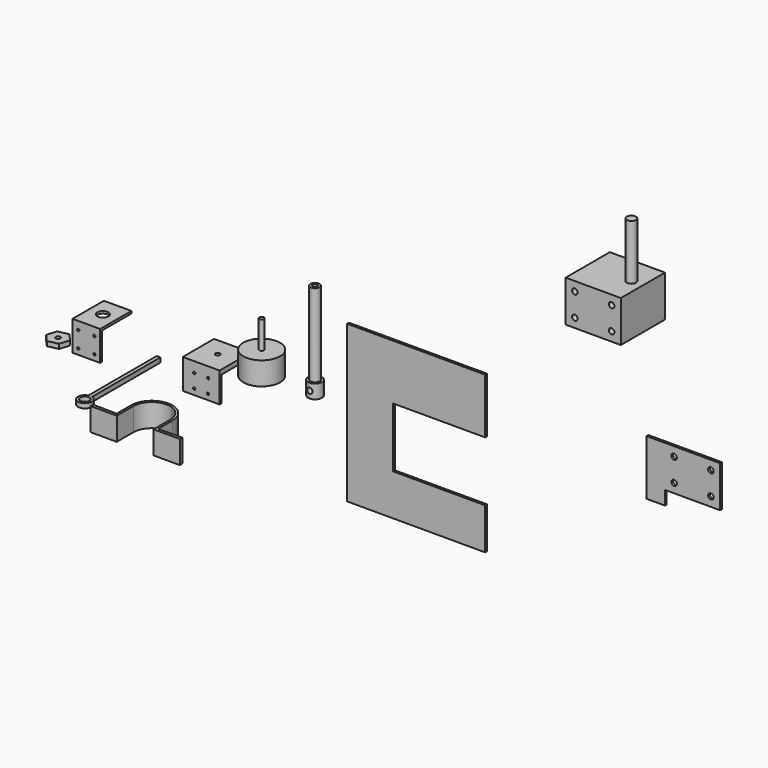
from build123d import *

# Parameters (mm, degrees)
F0_R      = 2.5
F1_DEPTH  = 15
F2_R      = 5
F2_R_2    = 2.5
F3_DEPTH  = 90
F5_R      = 3
F6_DEPTH  = 15.001
F0_R_2    = 20
F7_DEPTH  = 25
F8_R      = 2.5
F9_DEPTH  = 30
F0_W      = 40
F0_H      = 40
F10_DEPTH = 5
F11_W     = 40
F11_H     = 2.5
F12_DEPTH = 32.5
F14_DEPTH = 2.5
F0_W_2    = 30
F0_R_3    = 6
F16_DEPTH = 2.5
F17_W     = 30
F17_H     = 2.5
F18_DEPTH = 32.5
F19_DEPTH = 5
F20_R     = 1.25
F21_DEPTH = 2.5
F22_R     = 1.25
F23_DEPTH = 2.5
F13_W     = 60
F13_H     = 45
F13_R     = 3
F24_DEPTH = 60
F25_R     = 5
F26_DEPTH = 60
F27_DEPTH = 2.5
F28_R     = 3
F29_DEPTH = 25
F0_R_4    = 5
F30_DEPTH = 5
F31_DEPTH = 25


with BuildPart() as f1:
    # F0 (on Top) → F1 (new body)
    with BuildSketch(Plane.XY):
        with BuildLine():
            ThreePointArc((0, 7.5), (-5.3033008589, -5.3033008589), (7.5, 0))
            ThreePointArc((7.5, 0), (5.3033008589, 5.3033008589), (0, 7.5))
        make_face()
        Circle(F0_R, mode=Mode.SUBTRACT)
    extrude(amount=F1_DEPTH)

    # F2 (on face) → F3 (join)
    with BuildSketch(Plane.XY.offset(15)):
        Circle(F2_R)
        Circle(F2_R_2, mode=Mode.SUBTRACT)
    extrude(amount=F3_DEPTH)

    # F5 (on face) → F6 (cut, through all)
    with BuildSketch(Plane.XZ.offset(-7.5)):
        with Locations((0, 7.5)):
            Circle(F5_R)
    extrude(amount=F6_DEPTH, mode=Mode.SUBTRACT)


with BuildPart() as f7:
    # F0 (on Top) → F7 (new body)
    with BuildSketch(Plane.XY):
        with Locations((-57.9745993018, 0)):
            Circle(F0_R_2)
    extrude(amount=F7_DEPTH)

    # F8 (on face) → F9 (join)
    with BuildSketch(Plane.XY.offset(25)):
        with Locations((-57.9745993018, 0)):
            Circle(F8_R)
    extrude(amount=F9_DEPTH)


with BuildPart() as f10:
    # F0 (on Top) → F10 (new body)
    with BuildSketch(Plane.XY):
        with Locations((-105.7388707995, 0)):
            Rectangle(F0_W, F0_H)
        with Locations((-105.7388707995, 0)):
            Circle(F0_R, mode=Mode.SUBTRACT)
    extrude(amount=F10_DEPTH)

    # F11 (on face) → F12 (join)
    with BuildSketch(Plane.XY.offset(5)):
        with Locations((-105.7388707995, -21.25)):
            Rectangle(F11_W, F11_H)
    extrude(amount=-F12_DEPTH)

    # F20 (on face) → F21 (cut, through all)
    with BuildSketch(Plane(origin=(0, -20, 0), x_dir=(-1, 0, 0), z_dir=(0, 1, 0))):
        with Locations((98.2388707995, -6.25)):
            Circle(F20_R)
        with Locations((113.2388707995, -6.25)):
            Circle(F20_R)
        with Locations((113.2388707995, -21.25)):
            Circle(F20_R)
        with Locations((98.2388707995, -21.25)):
            Circle(F20_R)
    extrude(amount=-F21_DEPTH, mode=Mode.SUBTRACT)


with BuildPart() as f14:
    # F13 (on Front) → F14 (new body)
    with BuildSketch(Plane.XZ):
        Polygon((186.8768878281, 81.5050628316), (36.8768878281, 81.5050628316), (36.8768878281, -88.4949371684), (186.8768878281, -88.4949371684), (186.8768878281, -43.4949371684), (86.8768878281, -43.4949371684), (86.8768878281, 21.5050628316), (186.8768878281, 21.5050628316), align=None)
    extrude(amount=F14_DEPTH)


with BuildPart() as f16:
    # F0 (on Top) → F16 (new body)
    with BuildSketch(Plane.XY):
        with Locations((-230.5557584763, 0)):
            Rectangle(F0_W_2, F0_H)
        with Locations((-230.5557584763, 0)):
            Circle(F0_R_3, mode=Mode.SUBTRACT)
    extrude(amount=F16_DEPTH)

    # F17 (on face) → F18 (join)
    with BuildSketch(Plane.XY.offset(2.5)):
        with Locations((-230.5557584763, -21.25)):
            Rectangle(F17_W, F17_H)
    extrude(amount=-F18_DEPTH)

    # F22 (on face) → F23 (cut, through all)
    with BuildSketch(Plane(origin=(0, -20, 0), x_dir=(-1, 0, 0), z_dir=(0, 1, 0))):
        with Locations((221.8057584763, -6.25)):
            Circle(F22_R)
        with Locations((221.8057584763, -23.75)):
            Circle(F22_R)
        with Locations((239.3057584763, -23.75)):
            Circle(F22_R)
        with Locations((239.3057584763, -6.25)):
            Circle(F22_R)
    extrude(amount=-F23_DEPTH, mode=Mode.SUBTRACT)


with BuildPart() as f19:
    # F0 (on Top) → F19 (new body)
    with BuildSketch(Plane.XY):
        Polygon((-222.9001823011, -69.3075905842), (-219.3971571383, -58.4452201324), (-227.0527333135, -49.9803261255), (-238.2113346515, -52.3778025704), (-241.7143598142, -63.2401730222), (-234.058783639, -71.7050670291), align=None)
        with Locations((-230.5557584763, -60.8426965773)):
            Circle(F0_R, mode=Mode.SUBTRACT)
    extrude(amount=F19_DEPTH)


with BuildPart() as f24:
    # F13 (on Front) → F24 (new body)
    with BuildSketch(Plane.XZ):
        with Locations((302.3541259766, 178.6684757471)):
            Rectangle(F13_W, F13_H)
        with Locations((282.3541259766, 166.1684757471)):
            Circle(F13_R, mode=Mode.SUBTRACT)
        with Locations((282.3541259766, 191.1684757471)):
            Circle(F13_R, mode=Mode.SUBTRACT)
        with Locations((322.3541259766, 166.1684757471)):
            Circle(F13_R, mode=Mode.SUBTRACT)
        with Locations((322.3541259766, 191.1684757471)):
            Circle(F13_R, mode=Mode.SUBTRACT)
    extrude(amount=-F24_DEPTH)

    # F25 (on face) → F26 (join)
    with BuildSketch(Plane.XY.offset(201.1684757471)):
        with Locations((319.8541259766, 30)):
            Circle(F25_R)
    extrude(amount=F26_DEPTH)


with BuildPart() as f27:
    # F15 (on face) → F27 (new body)
    with BuildSketch(Plane.XZ.offset(2.5)):
        Polygon((444.2156124115, 81.5050628316), (364.2156124115, 81.5050628316), (364.2156124115, 21.5050628316), (384.2156124115, 21.5050628316), (384.2156124115, 36.5050628316), (444.2156124115, 36.5050628316), align=None)
    extrude(amount=F27_DEPTH)

    # F28 (on face) → F29 (cut)
    with BuildSketch(Plane.XZ.offset(5)):
        with Locations((394.2156124115, 71.5050628316)):
            Circle(F28_R)
        with Locations((394.2156124115, 46.5050628316)):
            Circle(F28_R)
        with Locations((434.2156124115, 71.5050628316)):
            Circle(F28_R)
        with Locations((434.2156124115, 46.5050628316)):
            Circle(F28_R)
    extrude(amount=-F29_DEPTH, mode=Mode.SUBTRACT)


with BuildPart() as f30:
    # F0 (on Top) → F30 (new body)
    with BuildSketch(Plane.XY):
        with BuildLine():
            Line((-144.055913806, -35.0423544645), (-144.055913806, -127.8139383171))
            ThreePointArc((-144.055913806, -127.8139383171), (-142.055913806, -142.5423544645), (-140.055913806, -127.8139383171))
            Line((-140.055913806, -127.8139383171), (-140.055913806, -35.0423544645))
            Line((-140.055913806, -35.0423544645), (-142.055913806, -35.0423544645))
            Line((-142.055913806, -35.0423544645), (-144.055913806, -35.0423544645))
        make_face()
        with Locations((-142.055913806, -135.0423544645)):
            Circle(F0_R_4, mode=Mode.SUBTRACT)
    extrude(amount=F30_DEPTH)


with BuildPart() as f31:
    # F0 (on Top) → F31 (new body)
    with BuildSketch(Plane.XY):
        with BuildLine():
            Line((-35.4745993018, -168.9512616546), (-35.4745993018, -149.3839472532))
            ThreePointArc((-35.4745993018, -149.3839472532), (-57.9745993018, -126.8839472532), (-80.4745993018, -149.3839472532))
            Line((-80.4745993018, -149.3839472532), (-80.4745993018, -168.9512616546))
            Line((-80.4745993018, -168.9512616546), (-106.4492836595, -168.4517562389))
            Line((-106.4492836595, -168.4517562389), (-106.4492836595, -171.8839472532))
            Line((-106.4492836595, -171.8839472532), (-80.4745993018, -171.8839472532))
            Line((-80.4745993018, -171.8839472532), (-77.9745993018, -171.8839472532))
            Line((-77.9745993018, -171.8839472532), (-77.9745993018, -149.3839472532))
            ThreePointArc((-77.9745993018, -149.3839472532), (-69.5790343502, -133.0947763963), (-51.4408905811, -130.481284733))
            ThreePointArc((-51.4408905811, -130.481284733), (-41.6854284449, -137.7795122048), (-37.9745993018, -149.3839472532))
            Line((-37.9745993018, -149.3839472532), (-37.9745993018, -171.8839472532))
            Line((-37.9745993018, -171.8839472532), (-35.4745993018, -171.8839472532))
            Line((-35.4745993018, -171.8839472532), (-9.4999149442, -171.8839472532))
            Line((-9.4999149442, -171.8839472532), (-9.4999149442, -168.4517562389))
            Line((-9.4999149442, -168.4517562389), (-35.4745993018, -168.9512616546))
        make_face()
    extrude(amount=F31_DEPTH)


solid = Compound([f1.part, f7.part, f10.part, f14.part, f16.part, f19.part, f24.part, f27.part, f30.part, f31.part])
